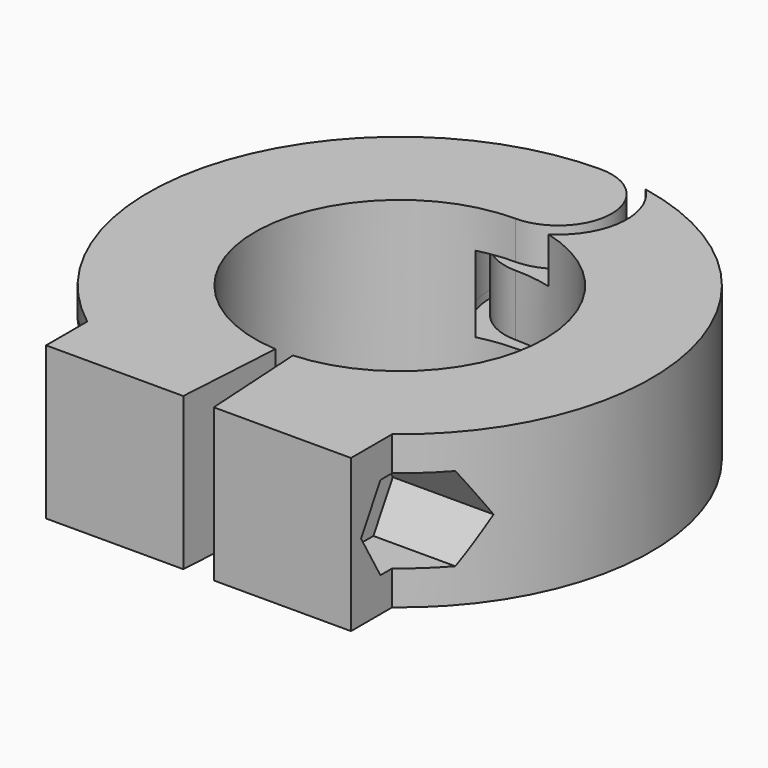
from build123d import *
from build123d import SkipClean  # not in build123d's __all__

# Parameters (mm, degrees)
F0_R           = 16.5
F0_R_2         = 9.5
F1_DEPTH       = 10
F3_DEPTH       = 2.5
F4_R           = 4.5
F4_R_2         = 1.5
F5_DEPTH       = 0.5
F7_DEPTH       = 2.5
F8_R           = 4.5
F8_R_2         = 1.5
F9_DEPTH       = 0.5
F10_R          = 2
F10_R_2        = 1.5
F11_DEPTH      = 4
F13_DEPTH      = 10
F15_DEPTH      = 10.001
F16_R          = 1.65
F17_DEPTH      = 20
F19_DEPTH      = 3
F19_DEPTH_BACK = 10
F20_R          = 3.75
F21_DEPTH      = 3
F21_DEPTH_BACK = 25


# Not quite as in the source:
# - after a boolean that leaves OpenCascade's solid faulty, fix() repairs it
# - a feature names something its author has since deleted; it is built from what else it names


with BuildPart() as f1:
    # F0 (on Top) → F1 (new body)
    with BuildSketch(Plane.XY):
        Circle(F0_R)
        Circle(F0_R_2, mode=Mode.SUBTRACT)
    extrude(amount=F1_DEPTH)

    # F2 (on face) → F3 (cut)
    with BuildSketch(Plane.XY.offset(10)):
        with BuildLine():
            ThreePointArc((0, 16.5), (3.5, 13), (0, 9.5))
            Line((0, 9.5), (0, 8.5))
            ThreePointArc((0, 8.5), (4.5, 13), (0, 17.5))
            Line((0, 17.5), (0, 16.5))
        make_face()
    extrude(amount=-F3_DEPTH, mode=Mode.SUBTRACT)

    # F4 (on face) → F5 (cut)
    with BuildSketch(Plane.XY.offset(7.5)):
        with Locations((0, 13)):
            Circle(F4_R)
        with Locations((0, 13)):
            Circle(F4_R_2, mode=Mode.SUBTRACT)
    extrude(amount=-F5_DEPTH, mode=Mode.SUBTRACT)

    # F6 (on face) → F7 (cut)
    with BuildSketch(Plane(origin=(0, 0, 0), x_dir=(1, 0, 0), z_dir=(0, 0, -1))):
        with BuildLine():
            ThreePointArc((0, -9.5), (3.5, -13), (0, -16.5))
            Line((0, -16.5), (0, -17.5))
            ThreePointArc((0, -17.5), (4.5, -13), (0, -8.5))
            Line((0, -8.5), (0, -9.5))
        make_face()
    extrude(amount=-F7_DEPTH, mode=Mode.SUBTRACT)

    # F8 (on face) → F9 (cut)
    with BuildSketch(Plane(origin=(0, 0, 2.5), x_dir=(1, 0, 0), z_dir=(0, 0, -1))):
        with Locations((0, -13)):
            Circle(F8_R)
        with Locations((0, -13)):
            Circle(F8_R_2, mode=Mode.SUBTRACT)
    extrude(amount=-F9_DEPTH, mode=Mode.SUBTRACT)

    # F10 (on face) → F11 (cut, through all)
    with BuildSketch(Plane(origin=(0, 0, 3), x_dir=(1, 0, 0), z_dir=(0, 0, -1))):
        with BuildLine():
            ThreePointArc((0, -16.5), (-3.5, -13), (0, -9.5))
            ThreePointArc((0, -9.5), (-1.2089410497, -9.4227629461), (-2.3982241951, -9.1923076923))
            ThreePointArc((-2.3982241951, -9.1923076923), (-4.472783282, -12.5058242088), (-3.171619712, -16.1923076923))
            ThreePointArc((-3.171619712, -16.1923076923), (-1.5932550136, -16.4228967744), (0, -16.5))
        make_face()
        with Locations((0, -13)):
            Circle(F10_R)
        with Locations((0, -13)):
            Circle(F10_R_2, mode=Mode.SUBTRACT)
    with SkipClean():  # cleaning this boolean's faces spoils the solid; the shape is the same uncleaned
        extrude(amount=-F11_DEPTH, mode=Mode.SUBTRACT)

    # F12 (on face) → F13 (join, through all)
    with BuildSketch(Plane.XY.offset(10)):
        with BuildLine():
            Line((-10, -13.1244047484), (-10, -16.5))
            Line((-10, -16.5), (0, -16.5))
            ThreePointArc((0, -16.5), (-5.2771830389, -15.6333406275), (-10, -13.1244047484))
        make_face()
        with BuildLine():
            ThreePointArc((10, -13.1244047484), (5.2771830389, -15.6333406275), (0, -16.5))
            Line((0, -16.5), (10, -16.5))
            Line((10, -16.5), (10, -13.1244047484))
        make_face()
    extrude(amount=-F13_DEPTH)

    add(f1.part.fix(), mode=Mode.REPLACE)

    # F14 (on face) → F15 (cut, through all)
    with BuildSketch(Plane.XY.offset(10)):
        Polygon((1, -16.5), (0, 0), (-1, -16.5), align=None)
    extrude(amount=-F15_DEPTH, mode=Mode.SUBTRACT)

    # F16 (on face) → F17 (cut, through all)
    with BuildSketch(Plane(origin=(-10, 0, 0), x_dir=(0, -1, 0), z_dir=(-1, 0, 0))):
        with Locations((12.5, 5)):
            Circle(F16_R)
    extrude(amount=-F17_DEPTH, mode=Mode.SUBTRACT)

    # F18 (on face) → F19 (cut, two sides)
    with BuildSketch(Plane.YZ.offset(10)) as f19_sk:
        Polygon((-10.9122867597, 2.25), (-9.3245735195, 5), (-10.9122867597, 7.75), (-14.0877132403, 7.75), (-15.6754264805, 5), (-14.0877132403, 2.25), align=None)
    extrude(amount=-F19_DEPTH, mode=Mode.SUBTRACT)
    extrude(f19_sk.sketch, amount=F19_DEPTH_BACK, mode=Mode.SUBTRACT)

    # F20 (on face) → F21 (cut, two sides)
    with BuildSketch(Plane(origin=(-10, 0, 0), x_dir=(0, -1, 0), z_dir=(-1, 0, 0))) as f21_sk:
        with Locations((12.5, 5)):
            Circle(F20_R)
    extrude(amount=-F21_DEPTH, mode=Mode.SUBTRACT)
    extrude(f21_sk.sketch, amount=F21_DEPTH_BACK, mode=Mode.SUBTRACT)


solid = f1.part
